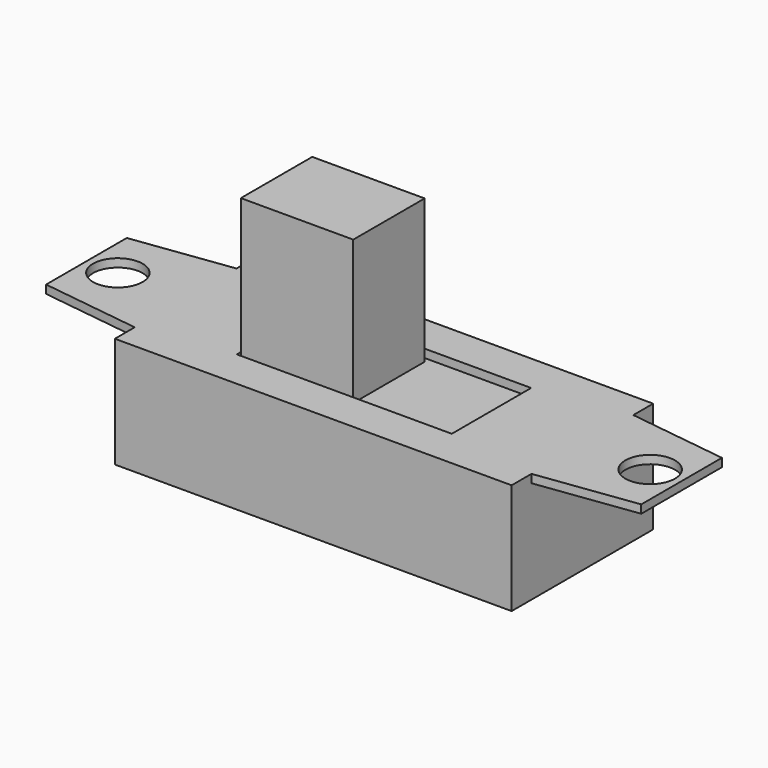
from build123d import *

# Parameters (mm, degrees)
F0_W      = 36
F0_H      = 10.7
F1_DEPTH  = 0.5
F2_W      = 24
F2_H      = 10.7
F3_DEPTH  = 6.2
F4_W      = 13
F4_H      = 6
F5_DEPTH  = 0.5
F6_W      = 6.8
F6_H      = 5.4
F7_DEPTH  = 8.7
F8_R      = 1.5
F9_DEPTH  = 0.5
F11_DEPTH = 0.5


# Not quite as in the source:
# - a pattern or mirror of a feature is missing from the dataset's text; its kind, count and spacing are read off the source's solid


with BuildPart() as f1:
    # F0 (on Top) → F1 (new body)
    with BuildSketch(Plane.XY):
        Rectangle(F0_W, F0_H)
    extrude(amount=F1_DEPTH)

    # F2 (on face) → F3 (join)
    with BuildSketch(Plane(origin=(0, 0, 0), x_dir=(1, 0, 0), z_dir=(0, 0, -1))):
        Rectangle(F2_W, F2_H)
    extrude(amount=F3_DEPTH)

    # F4 (on face) → F5 (cut)
    with BuildSketch(Plane.XY.offset(0.5)):
        Rectangle(F4_W, F4_H)
    extrude(amount=-F5_DEPTH, mode=Mode.SUBTRACT)

    # F6 (on face) → F7 (join)
    with BuildSketch(Plane.XY):
        with Locations((-3.1, 0)):
            Rectangle(F6_W, F6_H)
    extrude(amount=F7_DEPTH)

    # F8 (on face) → F9 (cut, through all)
    with BuildSketch(Plane.XY.offset(0.5)):
        with Locations((-16.1, 0)):
            Circle(F8_R)
        with Locations((16.1, 0)):
            Circle(F8_R)
    extrude(amount=-F9_DEPTH, mode=Mode.SUBTRACT)

    # F10 (on face) → F11 (cut, through all)
    with BuildSketch(Plane.XY.offset(0.5)):
        Polygon((-12, 3.85), (-12, 5.35), (-18, 5.35), (-18, 3.05), align=None)
        Polygon((-12, -3.85), (-18, -3.05), (-18, -5.35), (-12, -5.35), align=None)
    f11 = extrude(amount=-F11_DEPTH, mode=Mode.SUBTRACT)

    # F11_copies: F11 across plane
    add(f11.mirror(Plane(origin=(0, 0, 0), x_dir=(0, 0, 1), z_dir=(1, 0, 0))), mode=Mode.SUBTRACT)


solid = f1.part
